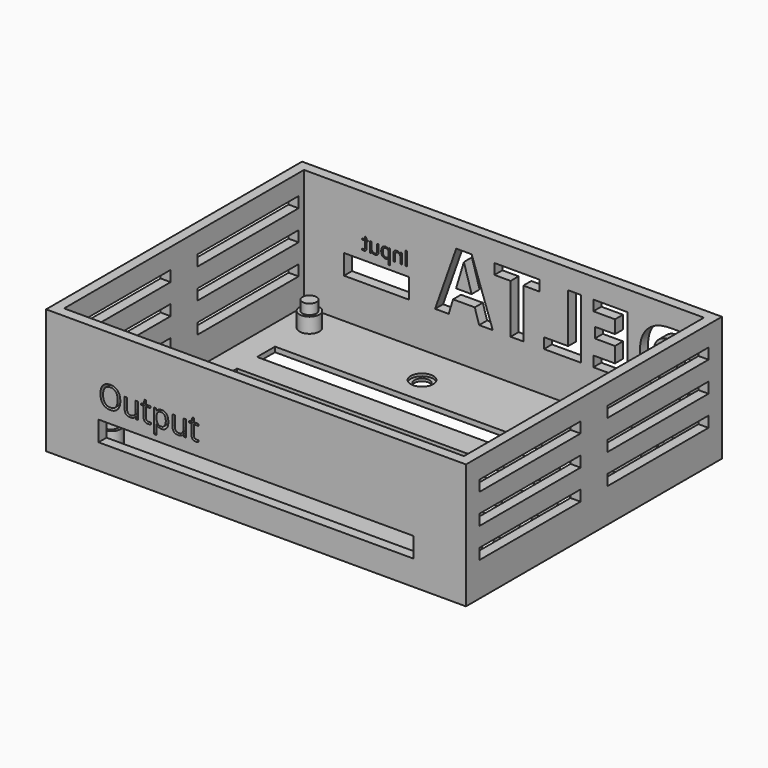
from build123d import *

# Parameters (mm, degrees)
F0_W           = 80
F0_H           = 60
F0_R           = 2
F0_R_2         = 2.5
F0_W_2         = 70
F0_H_2         = 4.5
F0_R_3         = 2.25
F1_DEPTH       = 1
F0_R_4         = 1.4
F2_DEPTH       = 4
F3_DEPTH       = 6
F0_W_3         = 84
F0_H_3         = 64
F4_DEPTH       = 25
F5_W           = 63
F5_H           = 4
F5_TEXT_SIZE   = 6.0618738644
F6_DEPTH       = 25
F7_W           = 13
F7_H           = 4
F7_TEXT_SIZE   = 16.7176942341
F7_TEXT_SIZE_2 = 3.83509323
F8_DEPTH       = 25
F9_W           = 25.2845270702
F9_H           = 2.1584379193
F10_DEPTH      = 89.4
F0_R_5         = 1.5
F11_DEPTH      = 0.5


# Not quite as in the source:
# - Text() gives the source's letters only with a copy of the font that has no kerning and outlines rounded to 1/6400 em; it was checked with that copy


with BuildPart() as f1:
    # F0 (on Top) → F1 (new body)
    with BuildSketch(Plane.XY):
        Rectangle(F0_W, F0_H)
        with Locations((-34.75, -24.8)):
            Circle(F0_R, mode=Mode.SUBTRACT)
        with Locations((34.75, -24.8)):
            Circle(F0_R_2, mode=Mode.SUBTRACT)
        with Locations((0, -14.25)):
            Rectangle(F0_W_2, F0_H_2, mode=Mode.SUBTRACT)
        with Locations((0, -4.75)):
            Rectangle(F0_W_2, F0_H_2, mode=Mode.SUBTRACT)
        with Locations((-34.75, 24.8)):
            Circle(F0_R, mode=Mode.SUBTRACT)
        with Locations((-10, 22)):
            Circle(F0_R_3, mode=Mode.SUBTRACT)
        with Locations((0, 4.75)):
            Rectangle(F0_W_2, F0_H_2, mode=Mode.SUBTRACT)
        with Locations((0, 14.25)):
            Rectangle(F0_W_2, F0_H_2, mode=Mode.SUBTRACT)
        with Locations((34.75, 24.8)):
            Circle(F0_R_2, mode=Mode.SUBTRACT)
    extrude(amount=F1_DEPTH)

    # F0 (on Top) → F2 (join)
    with BuildSketch(Plane.XY):
        with Locations((-34.75, -24.8)):
            Circle(F0_R)
        with Locations((-34.75, -24.8)):
            Circle(F0_R_4, mode=Mode.SUBTRACT)
        with Locations((-34.75, 24.8)):
            Circle(F0_R)
        with Locations((-34.75, 24.8)):
            Circle(F0_R_4, mode=Mode.SUBTRACT)
        with Locations((34.75, 24.8)):
            Circle(F0_R_2)
        with Locations((34.75, 24.8)):
            Circle(F0_R_4, mode=Mode.SUBTRACT)
        with Locations((34.75, -24.8)):
            Circle(F0_R_2)
        with Locations((34.75, -24.8)):
            Circle(F0_R_4, mode=Mode.SUBTRACT)
    extrude(amount=F2_DEPTH)

    # F0 (on Top) → F3 (join)
    with BuildSketch(Plane.XY):
        with Locations((-34.75, 24.8)):
            Circle(F0_R_4)
        with Locations((-34.75, -24.8)):
            Circle(F0_R_4)
        with Locations((34.75, -24.8)):
            Circle(F0_R_4)
    extrude(amount=F3_DEPTH)

    # F0 (on Top) → F4 (join)
    with BuildSketch(Plane.XY):
        Rectangle(F0_W_3, F0_H_3)
        Rectangle(F0_W, F0_H, mode=Mode.SUBTRACT)
    extrude(amount=F4_DEPTH)

    # F5 (on face) → F6 (cut)
    with BuildSketch(Plane.XZ.offset(32)):
        with Locations((0, 7)):
            Rectangle(F5_W, F5_H)
        with Locations((-31.5, 11.5004498512)):
            Text('Output', F5_TEXT_SIZE, font='Open Sans', text_align=(TextAlign.LEFT, TextAlign.BOTTOM))
    extrude(amount=-F6_DEPTH, mode=Mode.SUBTRACT)

    # F7 (on face) → F8 (cut)
    with BuildSketch(Plane(origin=(0, 32, 0), x_dir=(-1, 0, 0), z_dir=(0, 1, 0))):
        with Locations((25.5, 10.9730466524)):
            Rectangle(F7_W, F7_H)
        with Locations((-38.6188998818, 9.0614436194)):
            Text('DELTA', F7_TEXT_SIZE, font='Open Sans', font_style=FontStyle.BOLD, text_align=(TextAlign.LEFT, TextAlign.BOTTOM))
        with Locations((19, 14.7001165897)):
            Text('Input', F7_TEXT_SIZE_2, font='Open Sans', text_align=(TextAlign.LEFT, TextAlign.BOTTOM))
    extrude(amount=-F8_DEPTH, mode=Mode.SUBTRACT)

    # F9 (on face) → F10 (cut)
    with BuildSketch(Plane.YZ.offset(42)):
        with Locations((-16, 19.8767371476)):
            Rectangle(F9_W, F9_H)
        with Locations((-16, 13.8767371476)):
            Rectangle(F9_W, F9_H)
        with Locations((-16, 7.8767371476)):
            Rectangle(F9_W, F9_H)
        with Locations((16, 7.8767371476)):
            Rectangle(F9_W, F9_H)
        with Locations((16, 19.8767371476)):
            Rectangle(F9_W, F9_H)
        with Locations((16, 13.8767371476)):
            Rectangle(F9_W, F9_H)
    extrude(amount=-F10_DEPTH, mode=Mode.SUBTRACT)

    # F0 (on Top) → F11 (join)
    with BuildSketch(Plane.XY):
        with Locations((-10, 22)):
            Circle(F0_R_3)
        with Locations((-10, 22)):
            Circle(F0_R_5, mode=Mode.SUBTRACT)
    extrude(amount=F11_DEPTH)


solid = f1.part
